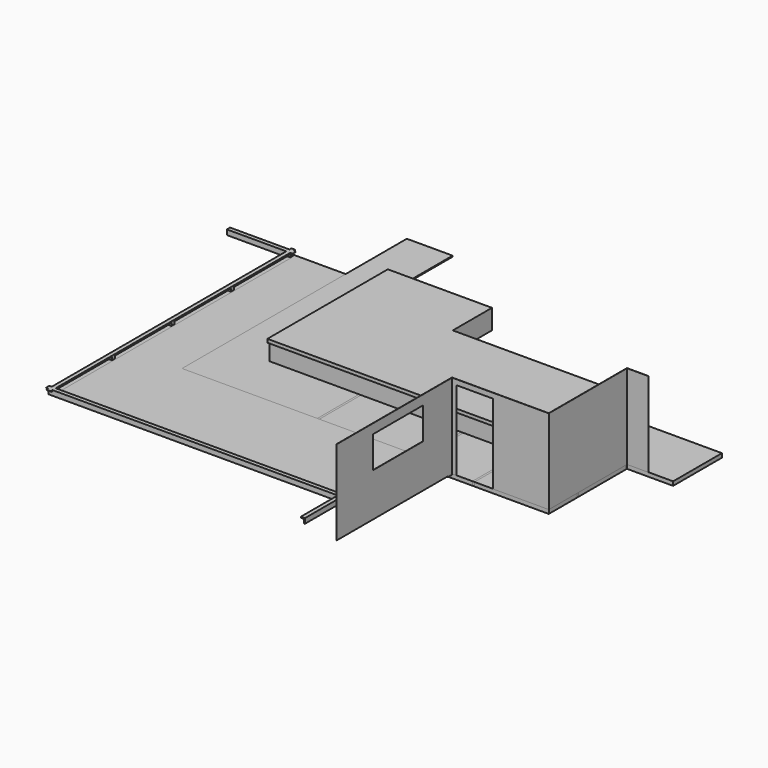
from build123d import *

# Parameters (mm, degrees)
F1_DEPTH  = 85
F3_DEPTH  = 410
F5_DEPTH  = 25
F7_DEPTH  = 25
F9_DEPTH  = 75
F10_W     = 25
F10_H     = 1300
F11_DEPTH = 100
F12_W     = 800
F12_H     = 75
F12_W_2   = 100
F12_H_2   = 60
F12_W_3   = 75
F12_H_3   = 3430
F12_W_4   = 60
F12_H_4   = 100
F13_DEPTH = 25
F15_DEPTH = 25
F16_SIZE  = 24.99999
F18_DEPTH = 25
F20_DEPTH = 2110
F21_W     = 3000
F21_H     = 1520
F22_DEPTH = 100
F23_W     = 50
F23_H     = 1480
F24_DEPTH = 100
F23_W_2   = 1850
F23_H_2   = 50
F23_H_3   = 1300
F25_W     = 1850
F25_H     = 1455
F26_DEPTH = 100
F25_H_2   = 880
F25_W_2   = 1410
F25_H_3   = 1480
F25_W_3   = 2500
F25_H_4   = 1300
F27_W     = 910
F27_H     = 1980
F28_DEPTH = 5
F29_W     = 1560
F29_H     = 790
F30_DEPTH = 5


# Not quite as in the source:
# - a fillet or chamfer is up to 0.001 mm smaller than in the source, because OpenCascade refuses the exact size


with BuildPart() as f1:
    # F0 (on Top) → F1 (new body)
    with BuildSketch(Plane.XY):
        Polygon((3755, 0), (0, 0), (0, 1220), (-2595, 1220), (-2595, -2530), (3755, -2530), align=None)
    extrude(amount=-F1_DEPTH)

    # F2 (on face) → F3 (join)
    with BuildSketch(Plane(origin=(0, 0, -85), x_dir=(1, 0, 0), z_dir=(0, 0, -1))):
        Polygon((-2565, 2500), (-2565, -1220), (0, -1220), (0, 0), (3725, 0), (3725, 2500), align=None)
    extrude(amount=F3_DEPTH)


with BuildPart() as f5:
    # F4 (on face) → F5 (new body)
    with BuildSketch(Plane(origin=(0, 0, -495), x_dir=(1, 0, 0), z_dir=(0, 0, -1))):
        Polygon((-2565, -3200), (-2565, 2500), (1875, 2500), (1875, 3800), (-3705, 3800), (-3705, -3200), align=None)
    extrude(amount=F5_DEPTH)


with BuildPart() as f7:
    # F6 (on face) → F7 (new body)
    with BuildSketch(Plane.XY.offset(-495)):
        Polygon((3165, -3980), (2215, -3980), (2215, -6110), (-4960, -6110), (-4960, 1295), (-6565, 1295), (-6565, 1170), (-5085, 1170), (-5085, -6235), (2340, -6235), (2340, -4105), (3165, -4105), align=None)
    extrude(amount=-F7_DEPTH)

    # F8 (on face) → F9 (join)
    with BuildSketch(Plane.XY.offset(-495)):
        Polygon((3165, -4005), (3140, -4005), (3140, -4080), (2340, -4080), (2340, -4005), (2240, -4005), (2240, -4105), (2315, -4105), (2315, -6135), (2240, -6135), (2240, -6210), (508.75, -6210), (508.75, -6135), (408.75, -6135), (408.75, -6210), (-1322.5, -6210), (-1322.5, -6135), (-1422.5, -6135), (-1422.5, -6210), (-3153.75, -6210), (-3153.75, -6135), (-3253.75, -6135), (-3253.75, -6210), (-4985, -6210), (-4985, -6135), (-5060, -6135), (-5060, -4383.75), (-4985, -4383.75), (-4985, -4283.75), (-5060, -4283.75), (-5060, -2532.5), (-4985, -2532.5), (-4985, -2432.5), (-5060, -2432.5), (-5060, -681.25), (-4985, -681.25), (-4985, -581.25), (-5060, -581.25), (-5060, 1170), (-4985, 1170), (-4985, 1270), (-5085, 1270), (-5085, 1195), (-6540, 1195), (-6540, 1270), (-6565, 1270), (-6565, 1170), (-5085, 1170), (-5085, -6235), (2340, -6235), (2340, -4105), (3165, -4105), align=None)
    extrude(amount=F9_DEPTH)

    # F10 (on face) → F11 (join)
    with BuildSketch(Plane.XY.offset(-420)):
        Polygon((3165, -4105), (3165, -4005), (3140, -4005), (3140, -4080), (2340, -4080), (2340, -4005), (2240, -4005), (2240, -4105), (2315, -4105), (2315, -6135), (2315, -6235), (2340, -6235), (2340, -4105), align=None)
        with Locations((2327.5, -6885)):
            Rectangle(F10_W, F10_H)
    extrude(amount=F11_DEPTH)

    # F12 (on face) → F13 (join)
    with BuildSketch(Plane.XY.offset(-320)):
        Polygon((2340, -4105), (3165, -4105), (3165, -4005), (3140, -4005), (3140, -4080), (2340, -4080), (2340, -4005), (2240, -4005), (2240, -4105), (2315, -4105), (2315, -7535), (2340, -7535), align=None)
        with Locations((2740, -4042.5)):
            Rectangle(F12_W, F12_H)
        with Locations((2290, -3975)):
            Rectangle(F12_W_2, F12_H_2)
        with Locations((2277.5, -5820)):
            Rectangle(F12_W_3, F12_H_3)
        with Locations((2210, -4055)):
            Rectangle(F12_W_4, F12_H_4)
    extrude(amount=F13_DEPTH)

    # F14 (on face) → F15 (join)
    with BuildSketch(Plane.XY.offset(-420)):
        Polygon((2315, -6235), (2315, -6135), (-4985, -6135), (-4985, 1170), (-4925, 1170), (-4925, 1270), (-4985, 1270), (-4985, 1330), (-5085, 1330), (-5085, 1270), (-6565, 1270), (-6565, 1170), (-5085, 1170), (-5085, -6135), (-5145, -6135), (-5145, -6235), (-5085, -6235), (-5085, -6295), (-4985, -6295), (-4985, -6235), align=None)
    extrude(amount=F15_DEPTH)

    # F16 (size 25 in the source; OpenCascade refuses exactly that, so slightly less here)
    f16_edges = [f7.edges().sort_by_distance(p)[0] for p in [
        (2180, -4055, -320),
        (2290, -3945, -320),
        (-5035, -6295, -420),
        (-5145, -6185, -420),
        (-5035, 1330, -420),
        (-4925, 1220, -420),
    ]]
    chamfer(f16_edges, length=F16_SIZE)


with BuildPart() as f18:
    # F17 (on face) → F18 (new body)
    with BuildSketch(Plane.XY.offset(-495)):
        Polygon((-3705, -3800), (-3705, 1295), (-4960, 1295), (-4960, -6110), (2215, -6110), (2215, -3800), (1875, -3800), align=None)
    extrude(amount=-F18_DEPTH)


with BuildPart() as f20:
    # F19 (on face) → F20 (new body)
    with BuildSketch(Plane.XY.offset(-495)):
        Polygon((3165, -3980), (3165, -7580), (3170, -7580), (3170, -3985), (5580, -3985), (5580, -1550), (6110, -1550), (6110, -1545), (5575, -1545), (5575, -3980), align=None)
    extrude(amount=F20_DEPTH)

    # F27 (on face) → F28 (cut, through all)
    with BuildSketch(Plane(origin=(0, -3980, 0), x_dir=(-1, 0, 0), z_dir=(0, 1, 0))):
        with Locations((-3730, 495)):
            Rectangle(F27_W, F27_H)
    extrude(amount=-F28_DEPTH, mode=Mode.SUBTRACT)

    # F29 (on face) → F30 (cut, through all)
    with BuildSketch(Plane(origin=(3165, 0, 0), x_dir=(0, -1, 0), z_dir=(-1, 0, 0))):
        with Locations((5670, 980)):
            Rectangle(F29_W, F29_H)
    extrude(amount=-F30_DEPTH, mode=Mode.SUBTRACT)


with BuildPart() as f22:
    # F21 (on face) → F22 (new body)
    with BuildSketch(Plane(origin=(0, 0, -495), x_dir=(1, 0, 0), z_dir=(0, 0, -1))):
        with Locations((5225, 785)):
            Rectangle(F21_W, F21_H)
    extrude(amount=F22_DEPTH)


with BuildPart() as f24:
    # F23 (on face) → F24 (new body)
    with BuildSketch(Plane.XY.offset(-495)):
        with Locations((2240, -3240)):
            Rectangle(F23_W, F23_H)
    extrude(amount=-F24_DEPTH)


with BuildPart() as f24b:
    # F23 (on face) → F24, piece 2 (new body)
    with BuildSketch(Plane.XY.offset(-495)):
        with Locations((4650, -1570)):
            Rectangle(F23_W_2, F23_H_2)
    extrude(amount=-F24_DEPTH)


with BuildPart() as f24c:
    # F23 (on face) → F24, piece 3 (new body)
    with BuildSketch(Plane.XY.offset(-495)):
        Polygon((3725, -3050), (3725, -2500), (3675, -2500), (3675, -3980), (3725, -3980), (3725, -3100), align=None)
        with Locations((4650, -3075)):
            Rectangle(F23_W_2, F23_H_2)
    extrude(amount=-F24_DEPTH)


with BuildPart() as f24d:
    # F23 (on face) → F24, piece 4 (new body)
    with BuildSketch(Plane.XY.offset(-495)):
        with Locations((-310, -3150)):
            Rectangle(F23_W, F23_H_3)
    extrude(amount=-F24_DEPTH)


with BuildPart() as f26:
    # F25 (on face) → F26 (new body)
    with BuildSketch(Plane.XY.offset(-495)):
        with Locations((4650, -2322.5)):
            Rectangle(F25_W, F25_H)
    extrude(amount=-F26_DEPTH)


with BuildPart() as f26b:
    # F25 (on face) → F26, piece 2 (new body)
    with BuildSketch(Plane.XY.offset(-495)):
        with Locations((4650, -3540)):
            Rectangle(F25_W, F25_H_2)
    extrude(amount=-F26_DEPTH)


with BuildPart() as f26c:
    # F25 (on face) → F26, piece 3 (new body)
    with BuildSketch(Plane.XY.offset(-495)):
        with Locations((2970, -3240)):
            Rectangle(F25_W_2, F25_H_3)
    extrude(amount=-F26_DEPTH)


with BuildPart() as f26d:
    # F25 (on face) → F26, piece 4 (new body)
    with BuildSketch(Plane.XY.offset(-495)):
        with Locations((965, -3150)):
            Rectangle(F25_W_3, F25_H_4)
    extrude(amount=-F26_DEPTH)


solid = Compound([f1.part, f5.part, f7.part, f18.part, f20.part, f22.part, f24.part, f24b.part, f24c.part, f24d.part, f26.part, f26b.part, f26c.part, f26d.part])
